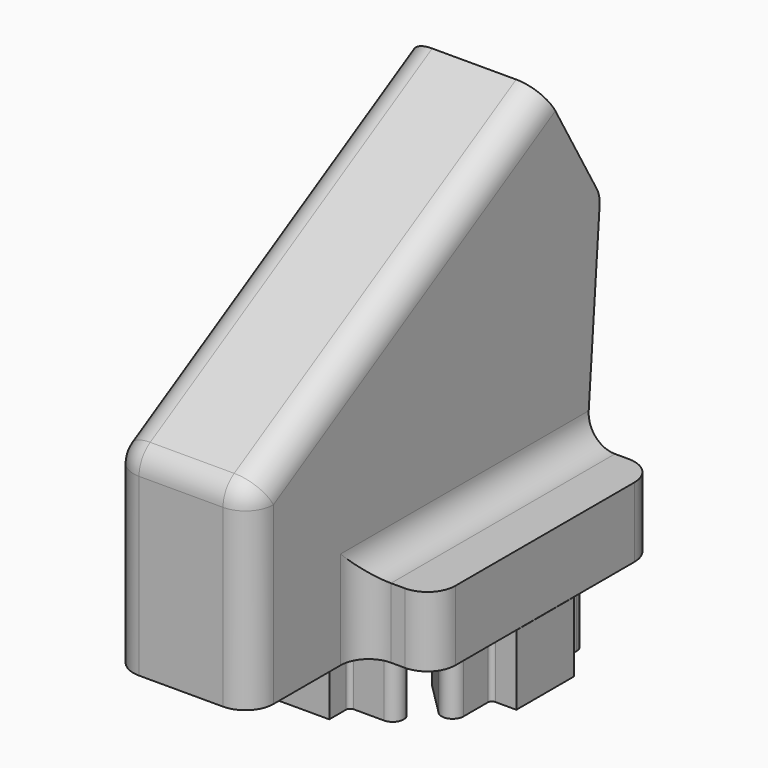
from build123d import *

# Parameters (mm, degrees)
F1_DEPTH = 5
F2_W     = 20
F2_H     = 20
F3_DEPTH = 5
F6_W     = 10
F6_H     = 10
F6_R     = 3
F9_DEPTH = 10
F10_R    = 2


with BuildPart() as f1:
    # F0 (on Top) → F1 (new body)
    with BuildSketch(Plane.XY):
        with BuildLine():
            Line((-11.8750007629, -7.425), (-12.575, -7.425))
            Line((-12.575, -7.425), (-13.375, -7.425))
            Line((-13.375, -7.425), (-13.375, -12.575))
            Line((-13.375, -12.575), (-12.575, -12.575))
            Line((-12.575, -12.575), (-11.8750007629, -12.575))
            ThreePointArc((-11.8750007629, -12.575), (-11.6628687671, -12.6628679271), (-11.5750007629, -12.8749998911))
            Line((-11.5750007629, -12.8749998911), (-11.5749999754, -15.0441214738))
            ThreePointArc((-11.5749999754, -15.0441214738), (-11.0934929218, -15.7647472802), (-10.2434566861, -15.5956644799))
            Line((-10.2434566861, -15.5956644799), (-7.9036796566, -13.2558874505))
            ThreePointArc((-7.9036796566, -13.2558874505), (-7.2533614014, -12.2826174011), (-7.0250000001, -11.1345671007))
            Line((-7.0250000001, -11.1345671007), (-7.0250000049, -8.8654328821))
            ThreePointArc((-7.0250000049, -8.8654328821), (-7.2533614085, -7.7173825884), (-7.9036796613, -6.7441125448))
            Line((-7.9036796613, -6.7441125448), (-10.2434566921, -4.404335514))
            ThreePointArc((-10.2434566921, -4.404335514), (-11.0934929289, -4.2352527142), (-11.5749999814, -4.9558785223))
            Line((-11.5749999814, -4.9558785223), (-11.5750007629, -7.1250001081))
            ThreePointArc((-11.5750007629, -7.1250001081), (-11.6628687668, -7.3371320726), (-11.8750007629, -7.425))
        make_face()
    extrude(amount=-F1_DEPTH)



with BuildPart() as f1b:
    # F0 (on Top) → F1, piece 2 (new body)
    with BuildSketch(Plane.XY):
        with BuildLine():
            Line((-0.8, -20), (-0.8, -19.2))
            Line((-0.8, -19.2), (-0.8, -18.5000007629))
            ThreePointArc((-0.8, -18.5000007629), (-0.7121320729, -18.2878687671), (-0.5000001089, -18.2000007629))
            Line((-0.5000001089, -18.2000007629), (1.6691214738, -18.1999999754))
            ThreePointArc((1.6691214738, -18.1999999754), (2.3897472802, -17.7184929218), (2.2206644799, -16.868456686))
            Line((2.2206644799, -16.868456686), (-0.1191125495, -14.5286796566))
            ThreePointArc((-0.1191125495, -14.5286796566), (-1.0923825989, -13.8783614014), (-2.2404328993, -13.6500000001))
            Line((-2.2404328993, -13.6500000001), (-4.5095671179, -13.6500000049))
            ThreePointArc((-4.5095671179, -13.6500000049), (-5.6576174116, -13.8783614085), (-6.6308874552, -14.5286796613))
            Line((-6.6308874552, -14.5286796613), (-8.970664486, -16.8684566921))
            ThreePointArc((-8.970664486, -16.8684566921), (-9.1397472858, -17.7184929288), (-8.4191214777, -18.1999999814))
            Line((-8.4191214777, -18.1999999814), (-6.2499998919, -18.2000007629))
            ThreePointArc((-6.2499998919, -18.2000007629), (-6.0378679274, -18.2878687668), (-5.95, -18.5000007629))
            Line((-5.95, -18.5000007629), (-5.95, -19.2))
            Line((-5.95, -19.2), (-5.95, -20))
            Line((-5.95, -20), (-0.8, -20))
        make_face()
    extrude(amount=-F1_DEPTH)


with BuildPart() as f1c:
    # F0 (on Top) → F1, piece 3 (new body)
    with BuildSketch(Plane.XY):
        with BuildLine():
            Line((3.4934566861, -4.4043355201), (1.1536796566, -6.7441125495))
            ThreePointArc((1.1536796566, -6.7441125495), (0.5033614014, -7.7173825989), (0.2750000001, -8.8654328993))
            Line((0.2750000001, -8.8654328993), (0.2750000049, -11.1345671179))
            ThreePointArc((0.2750000049, -11.1345671179), (0.5033614085, -12.2826174116), (1.1536796613, -13.2558874552))
            Line((1.1536796613, -13.2558874552), (3.4934566921, -15.595664486))
            ThreePointArc((3.4934566921, -15.595664486), (4.3434929289, -15.7647472858), (4.8249999814, -15.0441214777))
            Line((4.8249999814, -15.0441214777), (4.8250007629, -12.8749998919))
            ThreePointArc((4.8250007629, -12.8749998919), (4.9128687668, -12.6628679274), (5.1250007629, -12.575))
            Line((5.1250007629, -12.575), (5.825, -12.575))
            Line((5.825, -12.575), (6.625, -12.575))
            Line((6.625, -12.575), (6.625, -7.425))
            Line((6.625, -7.425), (5.825, -7.425))
            Line((5.825, -7.425), (5.1250007629, -7.425))
            ThreePointArc((5.1250007629, -7.425), (4.9128687671, -7.3371320729), (4.8250007629, -7.1250001089))
            Line((4.8250007629, -7.1250001089), (4.8249999754, -4.9558785262))
            ThreePointArc((4.8249999754, -4.9558785262), (4.3434929218, -4.2352527198), (3.4934566861, -4.4043355201))
        make_face()
    extrude(amount=-F1_DEPTH)


with BuildPart() as f1d:
    # F0 (on Top) → F1, piece 4 (new body)
    with BuildSketch(Plane.XY):
        with BuildLine():
            Line((-0.8, -1.4999992371), (-0.8, -0.8))
            Line((-0.8, -0.8), (-0.8, 0))
            Line((-0.8, 0), (-5.95, 0))
            Line((-5.95, 0), (-5.95, -0.8))
            Line((-5.95, -0.8), (-5.95, -1.4999992371))
            ThreePointArc((-5.95, -1.4999992371), (-6.0378679271, -1.7121312329), (-6.2499998911, -1.7999992371))
            Line((-6.2499998911, -1.7999992371), (-8.4191214738, -1.8000000246))
            ThreePointArc((-8.4191214738, -1.8000000246), (-9.1397472801, -2.2815070782), (-8.9706644799, -3.1315433139))
            Line((-8.9706644799, -3.1315433139), (-6.6308874505, -5.4713203434))
            ThreePointArc((-6.6308874505, -5.4713203434), (-5.6576174011, -6.1216385986), (-4.5095671007, -6.3499999999))
            Line((-4.5095671007, -6.3499999999), (-2.2404328821, -6.3499999951))
            ThreePointArc((-2.2404328821, -6.3499999951), (-1.0923825884, -6.1216385915), (-0.1191125448, -5.4713203387))
            Line((-0.1191125448, -5.4713203387), (2.220664486, -3.1315433079))
            ThreePointArc((2.220664486, -3.1315433079), (2.3897472858, -2.2815070711), (1.6691214777, -1.8000000186))
            Line((1.6691214777, -1.8000000186), (-0.5000001081, -1.7999992371))
            ThreePointArc((-0.5000001081, -1.7999992371), (-0.7121320726, -1.7121312332), (-0.8, -1.4999992371))
        make_face()
    extrude(amount=-F1_DEPTH)


with BuildPart() as f1_1:
    add(f1.part)

    add(f1b.part)  # F3 merges F1b

    add(f1c.part)  # F3 merges F1c

    add(f1d.part)  # F3 merges F1d
    # F2 (on face) → F3 (join)
    with BuildSketch(Plane.XY):
        with Locations((-3.3896967843, -10)):
            Rectangle(F2_W, F2_H)
    extrude(amount=F3_DEPTH)

    # F7: sweep along a path in F5
    with BuildLine(Plane.YZ.offset(-3.3896967843)) as f7_path:
        Line((-25, 0), (-25, 10.8014274722))
        Line((-25, 10.8014274722), (-1.3219409988, 24.4719612104))
    # F6 (on Top) → F7 (sweep)
    with BuildSketch(Plane.XY):
        with Locations((-3.3896967843, -25)):
            Rectangle(F6_W, F6_H)
        with Locations((-3.3896967843, -25)):
            Circle(F6_R, mode=Mode.SUBTRACT)
    sweep(path=f7_path.line, transition=Transition.RIGHT)

    # F8 (on face) → F9 (join)
    with BuildSketch(Plane.YZ.offset(1.6103032157)):
        Polygon((0, 5), (1.1780590012, 20.1418341915), (-20, 7.9146761262), (-20, 5), align=None)
    extrude(amount=-F9_DEPTH)

    # F10
    f10_edges = [f1_1.edges().sort_by_distance(p)[0] for p in [
        (6.610303, 0, 2.5),
        (6.610303, -20, 2.5),
        (-13.389697, 0, 2.5),
        (-13.389697, -20, 2.5),
        (-8.389697, -30, 6.844089),
        (1.610303, -30, 6.844089),
        (-8.389697, -16.91097, 21.245134),
        (1.610303, -16.91097, 21.245134),
        (-3.389697, -30, 13.688179),
        (-8.389697, -20, 2.5),
        (1.610303, -20, 2.5),
        (1.610303, -10, 5),
        (-8.389697, -10, 5),
        (-3.389697, 1.178059, 20.141834),
    ]]
    fillet(f10_edges, radius=F10_R)


solid = f1_1.part
